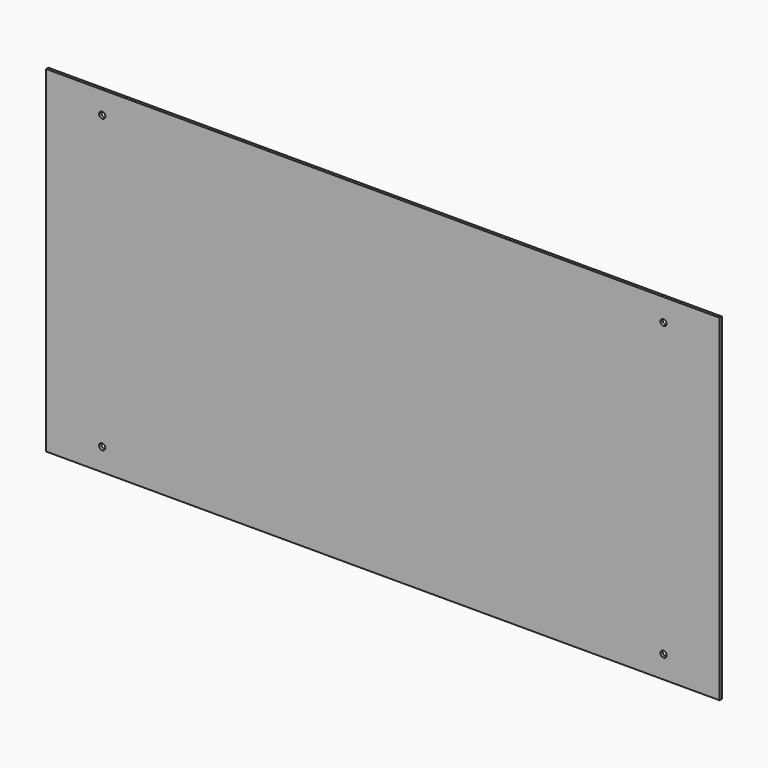
from build123d import *

# Parameters (mm, degrees)
F0_W     = 1200
F0_H     = 600
F0_R     = 5.5
F1_DEPTH = 5


# Not quite as in the source:
# - the program builds the solid bodies; features that only make, move or delete a surface that nothing else refers to are left out


with BuildPart() as f1:
    # F0 (on Front) → F1 (new body)
    with BuildSketch(Plane.XZ):
        with Locations((533.0324456096, 265.5700474977)):
            Rectangle(F0_W, F0_H)
        with Locations((33.0324456096, 5.5700474977)):
            Circle(F0_R, mode=Mode.SUBTRACT)
        with Locations((1033.0324456096, 5.5700474977)):
            Circle(F0_R, mode=Mode.SUBTRACT)
        with Locations((33.0324456096, 525.5700474977)):
            Circle(F0_R, mode=Mode.SUBTRACT)
        with Locations((1033.0324456096, 525.5700474977)):
            Circle(F0_R, mode=Mode.SUBTRACT)
    extrude(amount=F1_DEPTH)


solid = f1.part
